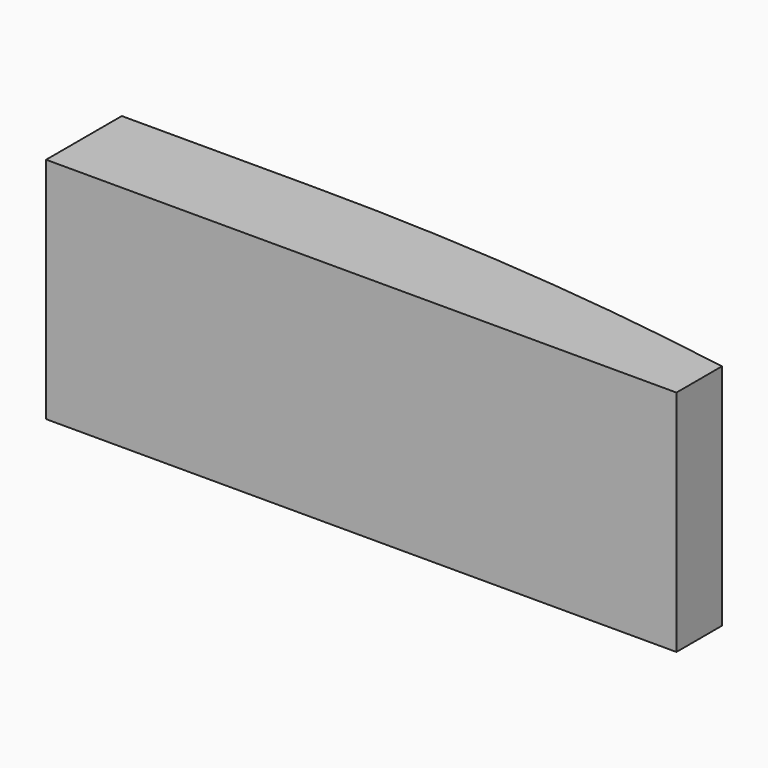
from build123d import *

# Parameters (mm, degrees)
F0_W        = 30.988
F0_H        = 11.2268
F1_DEPTH    = 1.857375
F3_T1_DEPTH = 119.4307056724
F2_W        = 30.988
F2_H        = 11.2268
F4_DEPTH    = 2.794


# Not quite as in the source:
# - a fillet or chamfer that OpenCascade refuses, or shapes differently, is made with other operations: its cross-section is extruded or revolved along the edge and cut away or added


with BuildPart() as f1:
    # F0 (on Front) → F1 (new body)
    with BuildSketch(Plane.XZ):
        with Locations((15.494, 5.6134)):
            Rectangle(F0_W, F0_H)
    extrude(amount=F1_DEPTH)

    # F3: fillet of radius 127 on 1 edges, made by hand

    # F3_s2 → F3_t1 (cut)
    with BuildSketch(Plane.XY.offset(-54.1019528362)):
        with BuildLine():
            ThreePointArc((30.988, -1.857375), (20.2073897896, -0.4651957464), (9.3472188655, 0))
            Line((9.3472188655, 0), (30.988, 0))
            Line((30.988, 0), (30.988, -1.857375))
        make_face()
    extrude(amount=F3_T1_DEPTH, mode=Mode.SUBTRACT)

    # F2 (on face) → F4 (join)
    with BuildSketch(Plane.XZ.offset(1.857375)):
        with Locations((15.494, 5.6134)):
            Rectangle(F2_W, F2_H)
    extrude(amount=F4_DEPTH)


solid = f1.part
